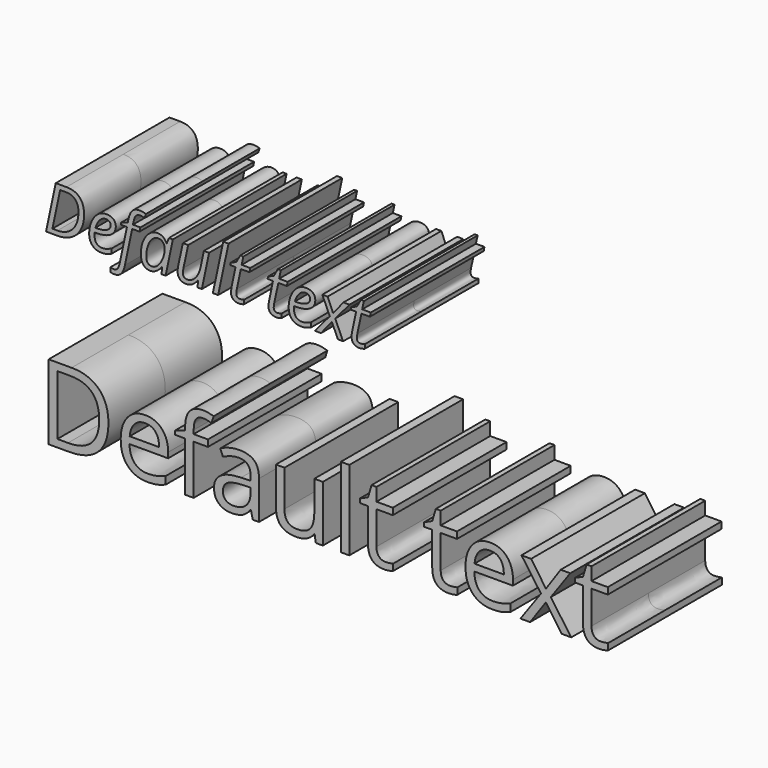
from build123d import *

# Parameters (mm, degrees)
F0_TEXT_SIZE   = 18.4367048658
F0_TEXT_SIZE_2 = 11.2779697196
F1_DEPTH       = 12.5


# Not quite as in the source:
# - Text() gives the source's letters only with a copy of the font that has no kerning and outlines rounded to 1/6400 em; it was checked with that copy


with BuildPart() as f1:
    # F0 (on Front) → F1 (new body, symmetric)
    with BuildSketch(Plane.XZ):
        with Locations((-54.0821310133, 0)):
            Text('Default text', F0_TEXT_SIZE, font='Open Sans', text_align=(TextAlign.LEFT, TextAlign.BOTTOM))
        with Locations((-53.2018654048, 32.7869653702)):
            Text('Default text', F0_TEXT_SIZE_2, font='Open Sans', font_style=FontStyle.ITALIC, text_align=(TextAlign.LEFT, TextAlign.BOTTOM))
    extrude(amount=F1_DEPTH, both=True)


solid = f1.part
